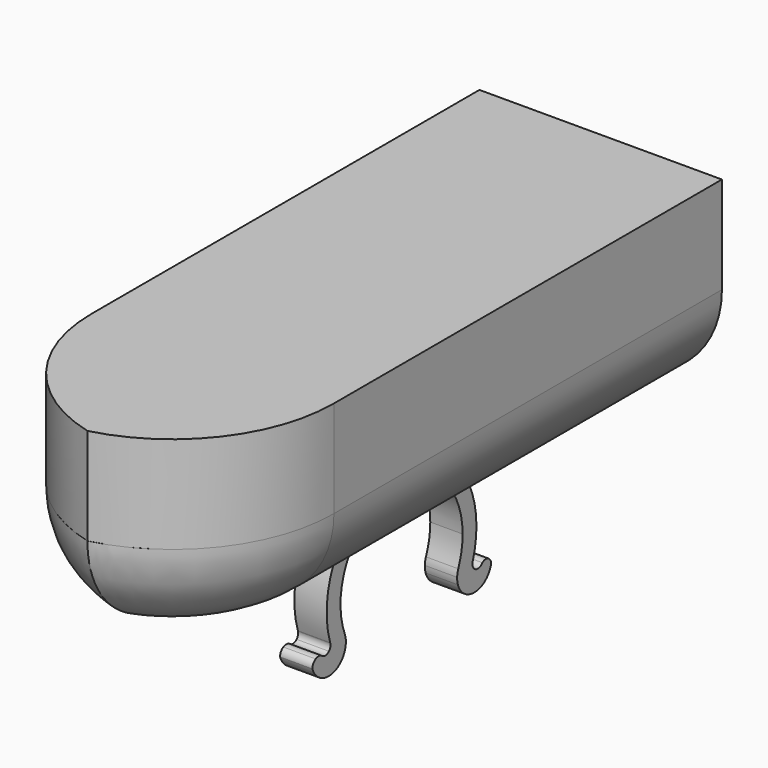
from build123d import *

# Parameters (mm, degrees)
F0_W        = 38.1
F0_H        = 101.6
F1_DEPTH    = 30.48
F2_T1_DEPTH = 157.48
F5_DEPTH    = 5.08
F6_T1_DEPTH = 114.3
F6_T4_ANGLE = 161.4904654603
F6_T6_ANGLE = 161.4904654612


# Not quite as in the source:
# - a fillet or chamfer that OpenCascade refuses, or shapes differently, is made with other operations: its cross-section is extruded or revolved along the edge and cut away or added


with BuildPart() as f1:
    # F0 (on Top) → F1 (new body)
    with BuildSketch(Plane.XY):
        with Locations((-7.3909840986, -8.8067197621)):
            Rectangle(F0_W, F0_H)
    extrude(amount=F1_DEPTH)

    # F2: fillet of radius 25.4 on 2 edges, made by hand

    # F2_s2 → F2_t1 (cut)
    with BuildSketch(Plane.XY.offset(-63.5)):
        with BuildLine():
            ThreePointArc((-13.7409840986, -59.6067197621), (4.2195281435, -52.1672320042), (11.6590159014, -34.2067197621))
            Line((11.6590159014, -34.2067197621), (11.6590159014, -59.6067197621))
            Line((11.6590159014, -59.6067197621), (-13.7409840986, -59.6067197621))
        make_face()
        with BuildLine():
            ThreePointArc((-26.4409840986, -34.2067197621), (-19.0014963408, -52.1672320042), (-1.0409840986, -59.6067197621))
            Line((-1.0409840986, -59.6067197621), (-26.4409840986, -59.6067197621))
            Line((-26.4409840986, -59.6067197621), (-26.4409840986, -34.2067197621))
        make_face()
    extrude(amount=F2_T1_DEPTH, mode=Mode.SUBTRACT)

    # F4 (on offset) → F5 (join)
    with BuildSketch(Plane.YZ.offset(-5.08)):
        with BuildLine():
            Line((-14.0174488836, -16.263814643), (-11.133858472, -16.263814643))
            ThreePointArc((-11.133858472, -16.263814643), (-2.2681486848, -0.0339935381), (11.991857098, -11.8093974888))
            ThreePointArc((11.991857098, -11.8093974888), (11.7754039507, -14.0775461736), (11.133858472, -16.263814643))
            Line((11.133858472, -16.263814643), (14.0174488836, -16.263814643))
            ThreePointArc((14.0174488836, -16.263814643), (14.5344751626, -14.0632247081), (14.7081849794, -11.8093974888))
            ThreePointArc((14.7081849794, -11.8093974888), (-2.2538272193, 2.7250776738), (-14.0174488836, -16.263814643))
        make_face()
        with BuildLine():
            ThreePointArc((-10.936740827, -17.3538234085), (-10.9902716166, -16.8006761373), (-11.133858472, -16.263814643))
            Line((-11.133858472, -16.263814643), (-14.0174488836, -16.263814643))
            ThreePointArc((-14.0174488836, -16.263814643), (-14.0054514358, -16.2990621553), (-13.9947204643, -16.3347156561))
            ThreePointArc((-13.9947204643, -16.3347156561), (-13.8183302749, -16.8476961899), (-13.6231437858, -17.3538234085))
            Line((-13.6231437858, -17.3538234085), (-10.936740827, -17.3538234085))
        make_face()
        with BuildLine():
            Line((14.0174488836, -16.263814643), (11.133858472, -16.263814643))
            ThreePointArc((11.133858472, -16.263814643), (10.9810910084, -16.799907635), (10.9185537399, -17.3538234085))
            Line((10.9185537399, -17.3538234085), (13.6231437858, -17.3538234085))
            ThreePointArc((13.6231437858, -17.3538234085), (13.781697315, -16.9470549808), (13.9281083774, -16.5357599818))
            ThreePointArc((13.9281083774, -16.5357599818), (13.9637636905, -16.3968256904), (14.0174488836, -16.263814643))
        make_face()
        with BuildLine():
            ThreePointArc((-11.1015096713, -18.4438321739), (-10.9743154761, -17.9056013647), (-10.936740827, -17.3538234085))
            Line((-10.936740827, -17.3538234085), (-13.6231437858, -17.3538234085))
            ThreePointArc((-13.6231437858, -17.3538234085), (-13.3861112566, -17.9038811268), (-13.1268801243, -18.4438321739))
            Line((-13.1268801243, -18.4438321739), (-11.1015096713, -18.4438321739))
        make_face()
        with BuildLine():
            Line((13.6231437858, -17.3538234085), (10.9185537399, -17.3538234085))
            ThreePointArc((10.9185537399, -17.3538234085), (10.9471844464, -17.9048318245), (11.0651192382, -18.4438321739))
            Line((11.0651192382, -18.4438321739), (13.1268801243, -18.4438321739))
            ThreePointArc((13.1268801243, -18.4438321739), (13.3861112566, -17.9038811268), (13.6231437858, -17.3538234085))
        make_face()
        with BuildLine():
            ThreePointArc((-13.6231437858, -17.3538234085), (-13.8183302749, -16.8476961899), (-13.9947204643, -16.3347156561))
            ThreePointArc((-13.9947204643, -16.3347156561), (-13.9894299583, -16.8803028031), (-14.2604863377, -17.3538234085))
            Line((-14.2604863377, -17.3538234085), (-13.6231437858, -17.3538234085))
        make_face()
        with BuildLine():
            ThreePointArc((-13.1268801243, -18.4438321739), (-13.3861112566, -17.9038811268), (-13.6231437858, -17.3538234085))
            Line((-13.6231437858, -17.3538234085), (-14.2604863377, -17.3538234085))
            ThreePointArc((-14.2604863377, -17.3538234085), (-14.9980791155, -17.659647367), (-15.7356718933, -17.3538234085))
            Line((-15.7356718933, -17.3538234085), (-16.868545512, -17.3538234085))
            ThreePointArc((-16.868545512, -17.3538234085), (-17.3451536393, -17.8087510018), (-17.5206139684, -18.4438321739))
            Line((-17.5206139684, -18.4438321739), (-13.1268801243, -18.4438321739))
        make_face()
        with BuildLine():
            ThreePointArc((-12.195911288, -20.0307388176), (-11.5329900367, -19.3170914758), (-11.1015096713, -18.4438321739))
            Line((-11.1015096713, -18.4438321739), (-13.1268801243, -18.4438321739))
            ThreePointArc((-13.1268801243, -18.4438321739), (-12.6862330658, -19.2518564902), (-12.195911288, -20.0307388176))
        make_face()
        with BuildLine():
            ThreePointArc((14.1034464611, -17.3538234085), (13.9336822531, -16.962387408), (13.9281083774, -16.5357599818))
            ThreePointArc((13.9281083774, -16.5357599818), (13.781697315, -16.9470549808), (13.6231437858, -17.3538234085))
            Line((13.6231437858, -17.3538234085), (14.1034464611, -17.3538234085))
        make_face()
        with BuildLine():
            Line((14.1034464611, -17.3538234085), (13.6231437858, -17.3538234085))
            ThreePointArc((13.6231437858, -17.3538234085), (13.3861112566, -17.9038811268), (13.1268801243, -18.4438321739))
            Line((13.1268801243, -18.4438321739), (17.526, -18.4438321739))
            Line((17.526, -18.4438321739), (17.526, -17.8258201323))
            ThreePointArc((17.526, -17.8258201323), (17.4025849977, -17.5677526977), (17.2126789083, -17.3538234085))
            Line((17.2126789083, -17.3538234085), (15.8839765936, -17.3538234085))
            ThreePointArc((15.8839765936, -17.3538234085), (14.9937115274, -17.8192920932), (14.1034464611, -17.3538234085))
        make_face()
        with BuildLine():
            Line((13.1268801243, -18.4438321739), (11.0651192382, -18.4438321739))
            ThreePointArc((11.0651192382, -18.4438321739), (11.4934563351, -19.3420700335), (12.1649032036, -20.0765514995))
            ThreePointArc((12.1649032036, -20.0765514995), (12.6722144503, -19.2757008789), (13.1268801243, -18.4438321739))
        make_face()
        with BuildLine():
            ThreePointArc((-12.195911288, -20.0307388176), (-12.6862330658, -19.2518564902), (-13.1268801243, -18.4438321739))
            Line((-13.1268801243, -18.4438321739), (-17.5206139684, -18.4438321739))
            ThreePointArc((-17.5206139684, -18.4438321739), (-15.2749066717, -20.6352919031), (-12.195911288, -20.0307388176))
        make_face()
        with BuildLine():
            Line((17.526, -18.4438321739), (13.1268801243, -18.4438321739))
            ThreePointArc((13.1268801243, -18.4438321739), (12.6722144503, -19.2757008789), (12.1649032036, -20.0765514995))
            ThreePointArc((12.1649032036, -20.0765514995), (15.2798483428, -20.6865502684), (17.526, -18.4438321739))
        make_face()
        with BuildLine():
            Line((-16.868545512, -17.3538234085), (-15.7356718933, -17.3538234085))
            ThreePointArc((-15.7356718933, -17.3538234085), (-15.7525545617, -17.3365203222), (-15.769031426, -17.3188303749))
            ThreePointArc((-15.769031426, -17.3188303749), (-16.3228921506, -17.2073853467), (-16.868545512, -17.3538234085))
        make_face()
        with BuildLine():
            ThreePointArc((17.2126789083, -17.3538234085), (16.548327751, -17.1094834068), (15.8839765936, -17.3538234085))
            Line((15.8839765936, -17.3538234085), (17.2126789083, -17.3538234085))
        make_face()
        with BuildLine():
            ThreePointArc((17.526, -18.4438321739), (17.5736704973, -18.1348261531), (17.526, -17.8258201323))
            Line((17.526, -17.8258201323), (17.526, -18.4438321739))
        make_face()
    extrude(amount=-F5_DEPTH)

    # F6: fillet of radius 15.24 on 4 edges, made by hand

    # F6_s2 → F6_t1 (cut)
    with BuildSketch(Plane.XZ.offset(-80.0932802379)):
        with BuildLine():
            ThreePointArc((11.6590159014, 15.24), (7.1953232467, 4.4636926547), (-3.5809840986, 0))
            Line((-3.5809840986, 0), (11.6590159014, 0))
            Line((11.6590159014, 0), (11.6590159014, 15.24))
        make_face()
        with BuildLine():
            ThreePointArc((-26.4409840986, 15.24), (-21.9772914439, 4.4636926547), (-11.2009840986, 0))
            Line((-11.2009840986, 0), (-26.4409840986, 0))
            Line((-26.4409840986, 0), (-26.4409840986, 15.24))
        make_face()
    extrude(amount=F6_T1_DEPTH, mode=Mode.SUBTRACT)

    # F6_s3 → F6_t4 (revolve, cut)
    with BuildSketch(Plane.XZ.offset(34.206719762)):
        with BuildLine():
            ThreePointArc((-3.5809840986, 0), (7.1953232467, 4.4636926547), (11.6590159014, 15.24))
            Line((11.6590159014, 15.24), (11.6590159014, 0))
            Line((11.6590159014, 0), (-3.5809840986, 0))
        make_face()
    revolve(axis=Axis((-13.7409840987, -34.206719762, 0), (0, 0, -1)), revolution_arc=F6_T4_ANGLE, mode=Mode.SUBTRACT)

    # F6_s5 → F6_t6 (revolve, cut)
    with BuildSketch(Plane(origin=(-10.402517324, -31.0726622139, 0), x_dir=(0, 0, 1), z_dir=(0.3174624617, 0.9482708397, 0))):
        with BuildLine():
            ThreePointArc((0, 20.0322145968), (4.4636926547, 30.8085219421), (15.24, 35.2722145968))
            Line((15.24, 35.2722145968), (0, 35.2722145968))
            Line((0, 35.2722145968), (0, 20.0322145968))
        make_face()
    revolve(axis=Axis((-1.0409840986, -34.2067197621, 0), (0, 0, -1)), revolution_arc=F6_T6_ANGLE, mode=Mode.SUBTRACT)


solid = f1.part
